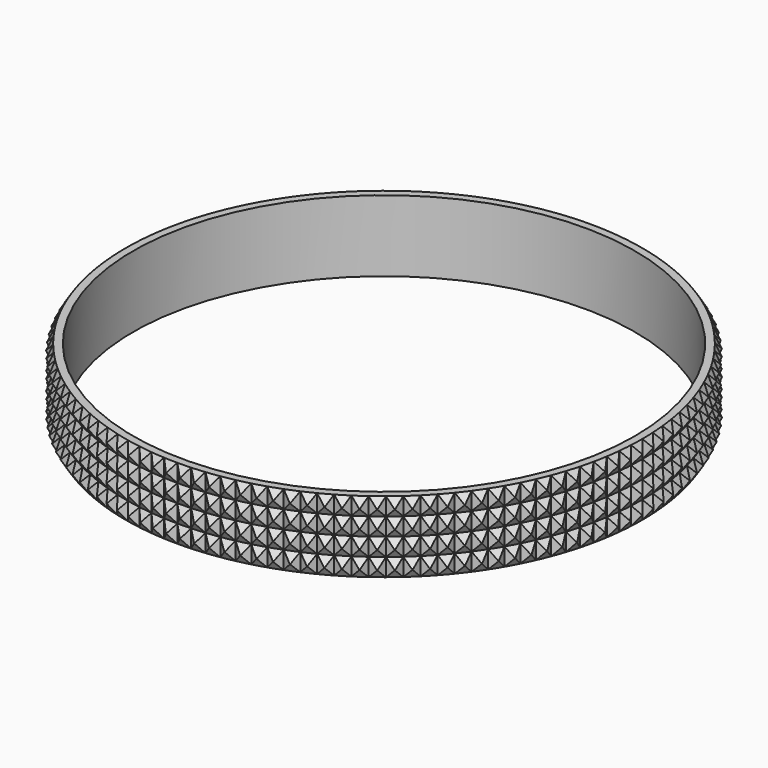
from build123d import *

# Parameters (mm, degrees)
F3_DEPTH        = 7.621
F3_COPIES_COUNT = 120


# Not quite as in the source:
# - a pattern or mirror of a feature is missing from the dataset's text; its kind, count and spacing are read off the source's solid


with BuildPart() as f1:
    # F0 (on Front) → F1 (revolve)
    with BuildSketch(Plane.XZ):
        Polygon((26.797, 7.62), (26.797, 0), (27.597, 0), (27.597, 1.905), (27.597, 3.81), (27.597, 5.715), (27.597, 7.62), align=None)
        Polygon((27.597, 1.905), (27.597, 0), (28.197, 0.9525), align=None)
        Polygon((28.197, 6.6675), (27.597, 7.62), (27.597, 5.715), align=None)
        Polygon((27.597, 3.81), (27.597, 1.905), (28.197, 2.8575), align=None)
        Polygon((28.197, 4.7625), (27.597, 5.715), (27.597, 3.81), align=None)
    revolve(axis=Axis((0, 0, 4.0968158282), (0, 0, 1)))

    # F2 (on Top) → F3 (cut, through all)
    with BuildSketch(Plane.XY):
        Polygon((0.7383644305, -28.197), (0, -27.597), (-0.7383644305, -28.197), align=None)
    f3 = extrude(amount=F3_DEPTH, mode=Mode.SUBTRACT)

    # F3_copies: F3 ×120 about axis
    f3_copies_axis = Axis((0, 0, 0), (0, 0, 1))
    for i in range(1, F3_COPIES_COUNT):
        add(f3.rotate(f3_copies_axis, i * 360 / F3_COPIES_COUNT), mode=Mode.SUBTRACT)


solid = f1.part
